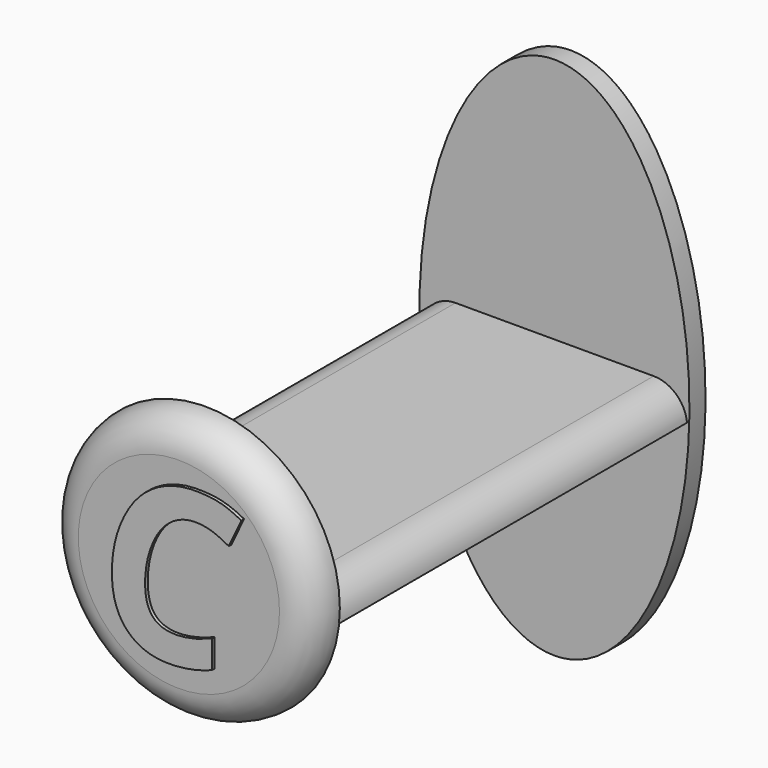
from build123d import *

# Parameters (mm, degrees)
F0_R         = 20
F1_DEPTH     = 5
F2_R         = 4.99999
F0_TEXT_SIZE = 32.6237938781
F4_DEPTH     = 5.5
F5_W         = 39.5
F5_H         = 4.5
F6_DEPTH     = 65
F7_T1_DEPTH  = 65
F10_DEPTH    = 3


# Not quite as in the source:
# - a fillet or chamfer that OpenCascade refuses, or shapes differently, is made with other operations: its cross-section is extruded or revolved along the edge and cut away or added
# - a fillet or chamfer is up to 0.001 mm smaller than in the source, because OpenCascade refuses the exact size
# - Text() gives the source's letters only with a copy of the font that has no kerning and outlines rounded to 1/6400 em; it was checked with that copy


with BuildPart() as f1:
    # F0 (on Front) → F1 (new body)
    with BuildSketch(Plane.XZ):
        Circle(F0_R)
        with BuildLine():
            add(Edge.make_bspline(
                [(5.0495509607, 7.689381468), (3.9510466512, 7.9901320678), (2.8652860112, 7.9901320678)],
                knots=[0, 0, 0, 1, 1, 1], degree=2))
            add(Edge.make_bspline(
                [(2.8652860112, 7.9901320678), (0.7651292803, 7.9901320678), (-0.9170350915, 6.700472716)],
                knots=[0, 0, 0, 1, 1, 1], degree=2))
            add(Edge.make_bspline(
                [(-0.9170350915, 6.700472716), (-2.5991994634, 5.4108133643), (-3.6186930221, 2.9028592099)],
                knots=[0, 0, 0, 1, 1, 1], degree=2))
            add(Edge.make_bspline(
                [(-3.6186930221, 2.9028592099), (-4.6381865808, 0.3949050555), (-4.6381865808, -2.4902617155)],
                knots=[0, 0, 0, 1, 1, 1], degree=2))
            add(Edge.make_bspline(
                [(-4.6381865808, -2.4902617155), (-4.6381865808, -5.1511399037), (-3.547328473, -6.4407992555)],
                knots=[0, 0, 0, 1, 1, 1], degree=2))
            add(Edge.make_bspline(
                [(-3.547328473, -6.4407992555), (-2.4564703652, -7.7304586072), (-0.06575797, -7.7304586072)],
                knots=[0, 0, 0, 1, 1, 1], degree=2))
            add(Edge.make_bspline(
                [(-0.06575797, -7.7304586072), (2.2586873438, -7.7304586072), (5.3171680199, -6.501968869)],
                knots=[0, 0, 0, 1, 1, 1], degree=2))
            Line((5.3171680199, -6.501968869), (5.3171680199, -10.6462101851))
            add(Edge.make_bspline(
                [(5.3171680199, -10.6462101851), (2.1516405201, -11.8746999233), (-1.054666722, -11.8746999233)],
                knots=[0, 0, 0, 1, 1, 1], degree=2))
            add(Edge.make_bspline(
                [(-1.054666722, -11.8746999233), (-5.0969586822, -11.8746999233), (-7.3449419791, -9.4916337298)],
                knots=[0, 0, 0, 1, 1, 1], degree=2))
            add(Edge.make_bspline(
                [(-7.3449419791, -9.4916337298), (-9.592925276, -7.1085675364), (-9.592925276, -2.7451351052)],
                knots=[0, 0, 0, 1, 1, 1], degree=2))
            add(Edge.make_bspline(
                [(-9.592925276, -2.7451351052), (-9.592925276, 1.4296910176), (-7.9362482431, 4.9418463273)],
                knots=[0, 0, 0, 1, 1, 1], degree=2))
            add(Edge.make_bspline(
                [(-7.9362482431, 4.9418463273), (-6.2795712102, 8.454001637), (-3.5065487306, 10.278895107)],
                knots=[0, 0, 0, 1, 1, 1], degree=2))
            add(Edge.make_bspline(
                [(-3.5065487306, 10.278895107), (-0.733526251, 12.1037885771), (2.8652860112, 12.1037885771)],
                knots=[0, 0, 0, 1, 1, 1], degree=2))
            add(Edge.make_bspline(
                [(2.8652860112, 12.1037885771), (4.8583959184, 12.1037885771), (6.4029286599, 11.7444170977)],
                knots=[0, 0, 0, 1, 1, 1], degree=2))
            add(Edge.make_bspline(
                [(6.4029286599, 11.7444170977), (7.9474614013, 11.3850456182), (9.7162827256, 10.4318191409)],
                knots=[0, 0, 0, 1, 1, 1], degree=2))
            Line((9.7162827256, 10.4318191409), (7.8353171098, 6.4455993264))
            add(Edge.make_bspline(
                [(7.8353171098, 6.4455993264), (6.1480552702, 7.3886308682), (5.0495509607, 7.689381468)],
                knots=[0, 0, 0, 1, 1, 1], degree=2))
        make_face(mode=Mode.SUBTRACT)
    extrude(amount=F1_DEPTH)

    # F2 (radius 5 in the source; OpenCascade refuses exactly that, so slightly less here)
    f2_edges = [f1.edges().sort_by_distance(p)[0] for p in [
        (-20, -5, 0),
    ]]
    fillet(f2_edges, radius=F2_R)

    # F0 (on Front) → F4 (join)
    with BuildSketch(Plane.XZ):
        with Locations((-11.5503529087, -11.5535594523)):
            Text('C', F0_TEXT_SIZE, font='Open Sans', font_style=FontStyle.BOLDITALIC, text_align=(TextAlign.LEFT, TextAlign.BOTTOM))
    extrude(amount=F4_DEPTH)

    # F5 (on offset) → F6 (join)
    with BuildSketch(Plane(origin=(0, 0, 0), x_dir=(-1, 0, 0), z_dir=(0, 1, 0))):
        with Locations((-0.0189123675, 0.13008592)):
            Rectangle(F5_W, F5_H)
    extrude(amount=F6_DEPTH)

    # F7: fillet of radius 5 on 2 edges, made by hand

    # F7_s2 → F7_t1 (cut)
    with BuildSketch(Plane.XZ.offset(-65)):
        with BuildLine():
            ThreePointArc((19.7689123675, -2.11991408), (18.1480771482, 1.0881851635), (14.793975182, 2.38008592))
            Line((14.793975182, 2.38008592), (14.793975182, 2.48008592))
            Line((14.793975182, 2.48008592), (19.7689123675, 2.48008592))
            Line((19.7689123675, 2.48008592), (19.8689123675, 2.38008592))
            ThreePointArc((19.8689123675, 2.38008592), (19.8689123675, 0.13008592), (19.8684111112, -2.10991408))
            Line((19.8684111112, -2.10991408), (19.7689123675, -2.11991408))
        make_face()
        with BuildLine():
            ThreePointArc((-19.7310876325, -2.11991408), (-18.1102524132, 1.0881851635), (-14.7561504469, 2.38008592))
            Line((-14.7561504469, 2.38008592), (-14.7561504469, 2.48008592))
            Line((-14.7561504469, 2.48008592), (-19.7310876325, 2.48008592))
            Line((-19.7310876325, 2.48008592), (-19.8310876325, 2.38008592))
            ThreePointArc((-19.8310876325, 2.38008592), (-19.8310876325, 0.13008592), (-19.8305863762, -2.10991408))
            Line((-19.8305863762, -2.10991408), (-19.7310876325, -2.11991408))
        make_face()
    extrude(amount=F7_T1_DEPTH, mode=Mode.SUBTRACT)

    # F9 (on offset) → F10 (join)
    with BuildSketch(Plane(origin=(0, 65, 0), x_dir=(-1, 0, 0), z_dir=(0, 1, 0))):
        with BuildLine():
            add(Edge.make_bspline(
                [(0, -39.1253754497), (34.8685415968, -39.1253754497), (17.4342707984, 19.5626877248), (0, 78.2507508993), (-17.4342707984, 19.5626877248), (-34.8685415968, -39.1253754497), (0, -39.1253754497)],
                knots=[0, 0, 0, 2.0943951024, 2.0943951024, 4.1887902048, 4.1887902048, 6.2831853072, 6.2831853072, 6.2831853072], degree=2, weights=[1, 0.5, 1, 0.5, 1, 0.5, 1]))
        make_face()
    extrude(amount=F10_DEPTH)


solid = f1.part
